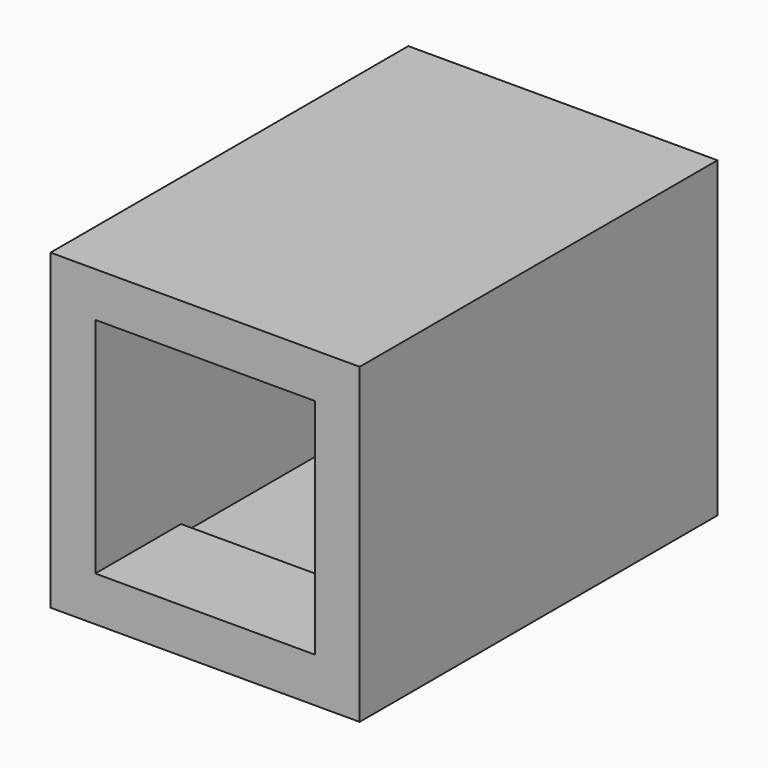
from build123d import *

# Parameters (mm, degrees)
F2_W     = 21.976557381
F2_H     = 31.7907221615
F3_DEPTH = 22.225
F1_W     = 15.621
F1_H     = 15.875
F1_H_2   = 0.635
F4_DEPTH = 28.6157221615
F5_DEPTH = 7.62


with BuildPart() as f3:
    # F2 (on Top) → F3 (new body)
    with BuildSketch(Plane.XY):
        with Locations((-0.0027786905, 15.8953610808)):
            Rectangle(F2_W, F2_H)
    extrude(amount=F3_DEPTH)

    # F1 (on Front) → F4 (cut, through all)
    with BuildSketch(Plane.XZ):
        with Locations((0, 11.1125)):
            Rectangle(F1_W, F1_H)
        with Locations((0, 2.8575)):
            Rectangle(F1_W, F1_H_2)
    extrude(amount=-F4_DEPTH, mode=Mode.SUBTRACT)

    # F1 (on Front) → F5 (join)
    with BuildSketch(Plane.XZ):
        with Locations((0, 2.8575)):
            Rectangle(F1_W, F1_H_2)
    extrude(amount=-F5_DEPTH)


solid = f3.part
